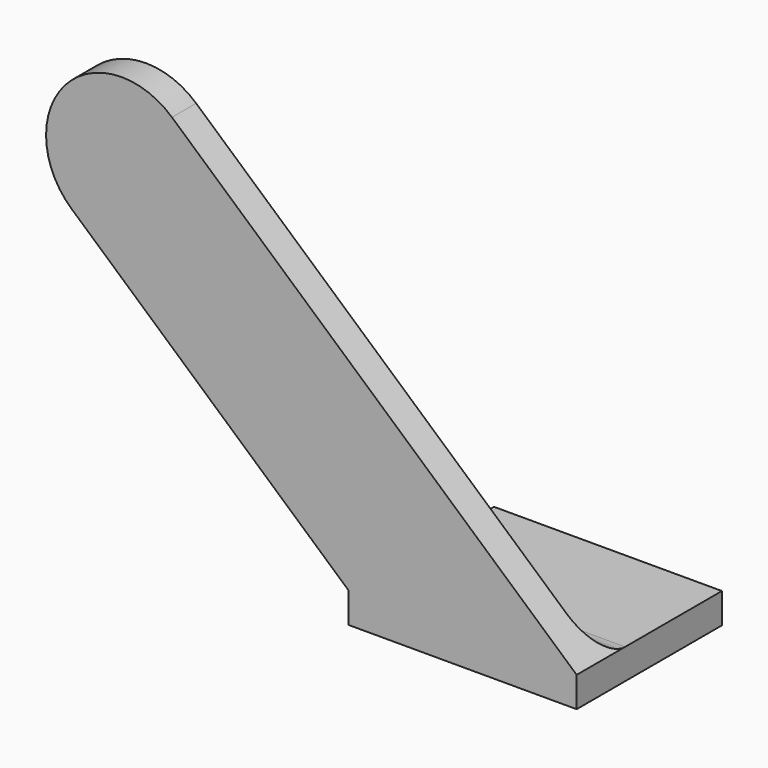
from build123d import *

# Parameters (mm, degrees)
F0_R          = 2.5
F1_DEPTH      = 2
F0_W          = 15.064
F0_H          = 2
F2_DEPTH      = 10
F2_DEPTH_BACK = 2
F3_DEPTH      = 2
F3_DEPTH_BACK = 2
F4_R          = 2


# Not quite as in the source:
# - ends of sketch curves that miss each other by under 0.0002 mm in the source are joined


with BuildPart() as f1:
    # F0 (on Front) → F1 (new body)
    with BuildSketch(Plane.XZ):
        with BuildLine():
            Line((30.0639452948, -20), (3.3191835885, 3.7393876913))
            ThreePointArc((3.3191835885, 3.7393876913), (-3.7393876913, 3.3191835885), (-3.3191835885, -3.7393876913))
            Line((-3.3191835885, -3.7393876913), (15, -20))
            Line((15, -20), (30.0639452948, -20))
        make_face()
        Circle(F0_R, mode=Mode.SUBTRACT)
    extrude(amount=F1_DEPTH)

    # F0 (on Front) → F2 (join, two sides)
    with BuildSketch(Plane.XZ) as f2_sk:
        with Locations((22.532, -21)):
            Rectangle(F0_W, F0_H)
    extrude(amount=-F2_DEPTH)
    extrude(f2_sk.sketch, amount=F2_DEPTH_BACK)

    # F0 (on Front) → F3 (join, two sides)
    with BuildSketch(Plane.XZ) as f3_sk:
        Circle(F0_R)
    extrude(amount=F3_DEPTH)
    extrude(f3_sk.sketch, amount=-F3_DEPTH_BACK)

    # F4
    f4_edges = [f1.edges().sort_by_distance(p)[0] for p in [
        (22.531973, 0, -20),
    ]]
    fillet(f4_edges, radius=F4_R)


solid = f1.part
